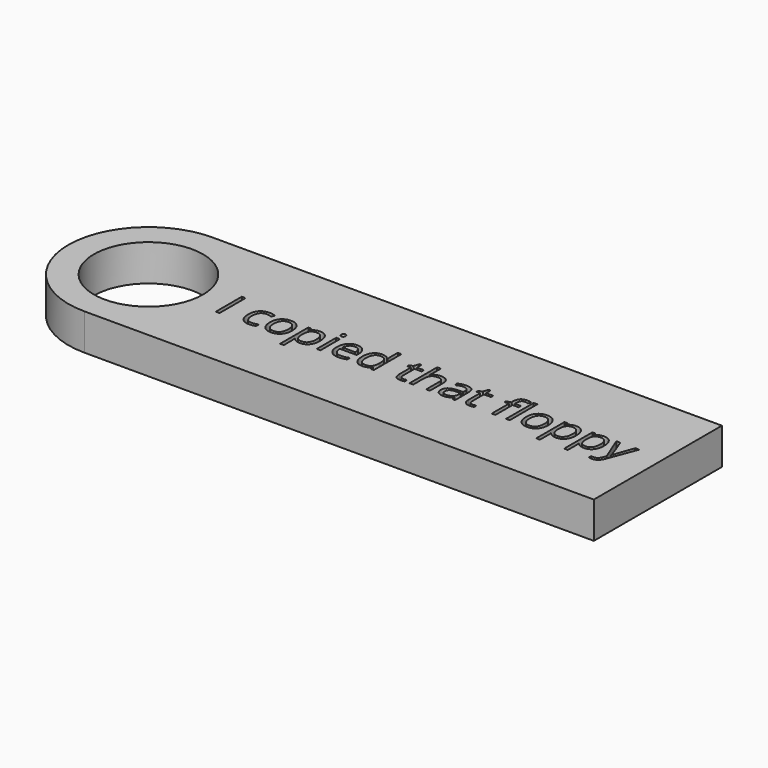
from build123d import *

# Parameters (mm, degrees)
F0_R         = 7.5
F1_DEPTH     = 5
F2_TEXT_SIZE = 6.25
F3_DEPTH     = 2.5


# Not quite as in the source:
# - Text() gives the source's letters only with a copy of the font that has no kerning and outlines rounded to 1/6400 em; it was checked with that copy


with BuildPart() as f1:
    # F0 (on Top) → F1 (new body)
    with BuildSketch(Plane.XY):
        with BuildLine():
            Line((39.9027594179, 15.3666207343), (39.9027594179, 37.3666207343))
            Line((39.9027594179, 37.3666207343), (-30.0972405821, 37.3666207343))
            ThreePointArc((-30.0972405821, 37.3666207343), (-41.0972405821, 26.3666207343), (-30.0972405821, 15.3666207343))
            Line((-30.0972405821, 15.3666207343), (39.9027594179, 15.3666207343))
        make_face()
        with Locations((-30.0972405821, 26.3666207343)):
            Circle(F0_R, mode=Mode.SUBTRACT)
    extrude(amount=F1_DEPTH)

    # F2 (on face) → F3 (cut)
    with BuildSketch(Plane.XY.offset(5)):
        with Locations((-19.6577405821, 24.1166207343)):
            Text('I copied that floppy', F2_TEXT_SIZE, font='Open Sans', text_align=(TextAlign.LEFT, TextAlign.BOTTOM))
    extrude(amount=-F3_DEPTH, mode=Mode.SUBTRACT)


solid = f1.part
